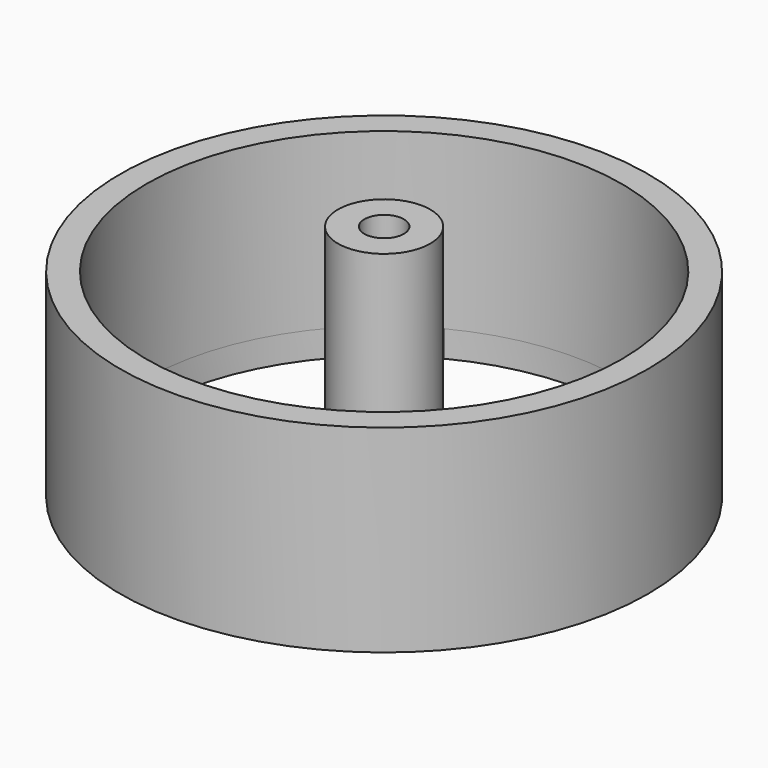
from build123d import *

# Parameters (mm, degrees)
F0_R     = 20
F1_DEPTH = 15
F2_R     = 18
F3_DEPTH = 13
F4_R     = 3.5
F4_R_2   = 1.5
F5_DEPTH = 16
F7_DEPTH = 2


with BuildPart() as f1:
    # F0 (on Top) → F1 (new body)
    with BuildSketch(Plane.XY):
        Circle(F0_R)
    extrude(amount=F1_DEPTH)

    # F2 (on face) → F3 (cut)
    with BuildSketch(Plane.XY.offset(15)):
        Circle(F2_R)
    extrude(amount=-F3_DEPTH, mode=Mode.SUBTRACT)

    # F4 (on face) → F5 (join)
    with BuildSketch(Plane.XY.offset(2)):
        Circle(F4_R)
        Circle(F4_R_2, mode=Mode.SUBTRACT)
    extrude(amount=F5_DEPTH)

    # F6 (on face) → F7 (cut)
    with BuildSketch(Plane(origin=(0, 0, 0), x_dir=(1, 0, 0), z_dir=(0, 0, -1))):
        with BuildLine():
            ThreePointArc((-1.9313093683, 2.9189114622), (-1.42176068, 3.1982177175), (-0.8730234102, 3.3893701664))
            Line((-0.8730234102, 3.3893701664), (-2.7039568663, 17.7957471679))
            ThreePointArc((-2.7039568663, 17.7957471679), (-10.7932215062, 14.4050813784), (-16.3196684485, 7.5939727238))
            Line((-16.3196684485, 7.5939727238), (-1.9313093683, 2.9189114622))
        make_face()
        with BuildLine():
            ThreePointArc((-3.3728571828, -0.9347911128), (-3.4810340129, -0.3638711329), (-3.4932616532, 0.2170783785))
            Line((-3.4932616532, 0.2170783785), (-17.7603299302, 2.927572505))
            ThreePointArc((-17.7603299302, 2.927572505), (-17.0353353821, -5.813548694), (-12.2653521367, -13.1742603953))
            Line((-12.2653521367, -13.1742603953), (-3.3728571828, -0.9347911128))
        make_face()
        with BuildLine():
            ThreePointArc((-0.1532310099, -3.4966441423), (-0.7296366559, -3.4231024452), (-1.285931023, -3.2552083503))
            Line((-1.285931023, -3.2552083503), (-8.2725306819, -15.9864078553))
            ThreePointArc((-8.2725306819, -15.9864078553), (0.2648052303, -17.9980520665), (8.7392639441, -15.7361134247))
            Line((8.7392639441, -15.7361134247), (-0.1532310099, -3.4966441423))
        make_face()
        with BuildLine():
            ThreePointArc((18, 0), (17.9164345956, 1.7324466465), (17.6665142908, 3.448807448))
            Line((17.6665142908, 3.448807448), (3.2781552106, -1.2262538137))
            ThreePointArc((3.2781552106, -1.2262538137), (3.0300937601, -1.7517225252), (2.6985125738, -2.2289077794))
            Line((2.6985125738, -2.2289077794), (12.6476247957, -12.8077159176))
            ThreePointArc((12.6476247957, -12.8077159176), (16.6080890882, -6.9405602683), (18, 0))
        make_face()
        with BuildLine():
            Line((2.1792423504, 17.8675936482), (2.1792423504, 2.7387776066))
            ThreePointArc((2.1792423504, 2.7387776066), (2.6023375887, 2.3404783858), (2.9537035127, 1.8776675848))
            Line((2.9537035127, 1.8776675848), (16.0891926827, 8.0708041))
            ThreePointArc((16.0891926827, 8.0708041), (10.3647576432, 14.7163785966), (2.1792423504, 17.8675936482))
        make_face()
    extrude(amount=-F7_DEPTH, mode=Mode.SUBTRACT)


solid = f1.part
